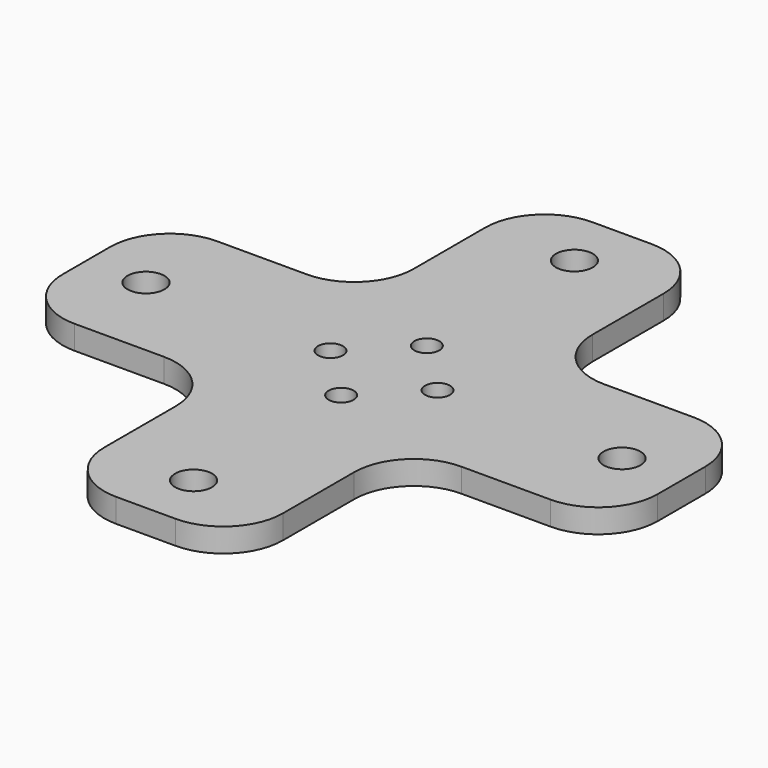
from build123d import *

# Parameters (mm, degrees)
F0_W            = 15
F0_H            = 17.5
F0_H_2          = 15
F0_W_2          = 17.5
F1_DEPTH        = 2
F2_R            = 1.05
F2_R_2          = 1.55
F3_DEPTH        = 25
F3_COPIES_COUNT = 4
F4_R            = 5


# Not quite as in the source:
# - a pattern or mirror of a feature is missing from the dataset's text; its kind, count and spacing are read off the source's solid


with BuildPart() as f1:
    # F0 (on Top) → F1 (new body)
    with BuildSketch(Plane.XY):
        with Locations((0, 16.25)):
            Rectangle(F0_W, F0_H)
        Rectangle(F0_W, F0_H_2)
        with Locations((-16.25, 0)):
            Rectangle(F0_W_2, F0_H_2)
        with Locations((16.25, 0)):
            Rectangle(F0_W_2, F0_H_2)
        with Locations((0, -16.25)):
            Rectangle(F0_W, F0_H)
    extrude(amount=F1_DEPTH)

    # F2 (on face) → F3 (cut)
    with BuildSketch(Plane.XY.offset(2)):
        with Locations((-4.5, 0)):
            Circle(F2_R)
        with Locations((-20, 0)):
            Circle(F2_R_2)
    f3 = extrude(amount=-F3_DEPTH, mode=Mode.SUBTRACT)

    # F3_copies: F3 ×4 about axis
    f3_copies_axis = Axis((0, 0, 0), (0, 0, 1))
    for i in range(1, F3_COPIES_COUNT):
        add(f3.rotate(f3_copies_axis, i * 360 / F3_COPIES_COUNT), mode=Mode.SUBTRACT)

    # F4
    f4_edges = [f1.edges().sort_by_distance(p)[0] for p in [
        (7.5, -25, 1),
        (-7.5, -25, 1),
        (-7.5, -7.5, 1),
        (-25, -7.5, 1),
        (-25, 7.5, 1),
        (-7.5, 7.5, 1),
        (-7.5, 25, 1),
        (7.5, 25, 1),
        (25, 7.5, 1),
        (7.5, 7.5, 1),
        (25, -7.5, 1),
        (7.5, -7.5, 1),
    ]]
    fillet(f4_edges, radius=F4_R)


solid = f1.part
